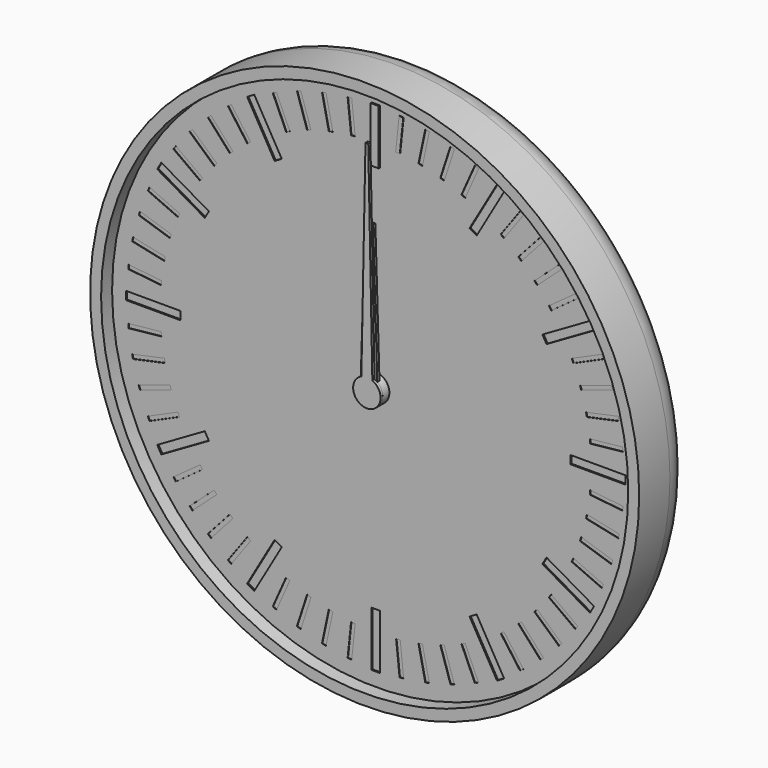
from build123d import *

# Parameters (mm, degrees)
F0_R      = 100
F1_DEPTH  = 24
F2_R      = 10
F3_T      = -4
F4_R      = 5
F4_R_2    = 3
F5_DEPTH  = 2
F6_DEPTH  = 19
F7_DEPTH  = 8
F9_DEPTH  = 4
F11_DEPTH = 4
F12_R     = 5
F12_R_2   = 3
F13_DEPTH = 2
F14_R     = 3
F15_DEPTH = 4
F17_DEPTH = 4
F18_R     = 3
F19_DEPTH = 2
F20_R     = 98
F20_R_2   = 5
F21_DEPTH = 1
F23_R     = 5
F23_R_2   = 3
F24_DEPTH = 2
F25_W     = 3
F25_H     = 20
F25_W_2   = 20
F25_H_2   = 3
F26_DEPTH = 0.5
F27_W     = 1.5
F27_H     = 12
F27_W_2   = 12
F27_H_2   = 1.5
F28_DEPTH = 0.2
F29_DEPTH = 1
F30_DEPTH = 0.4
F31_R     = 5
F31_R_2   = 3
F32_DEPTH = 5
F33_R     = 3
F34_DEPTH = 1
F36_DEPTH = 1


with BuildPart() as f1:
    # F0 (on Front) → F1 (new body)
    with BuildSketch(Plane.XZ):
        Circle(F0_R)
    extrude(amount=F1_DEPTH)

    # F2
    f2_edges = [f1.edges().sort_by_distance(p)[0] for p in [
        (-100, 0, 0),
    ]]
    fillet(f2_edges, radius=F2_R)

    # F3
    f3_openings = [f1.faces().sort_by_distance(p)[0] for p in [
        (0, -24, 0),
    ]]
    offset(amount=F3_T, openings=f3_openings)

    # F4 (on face) → F5 (join)
    with BuildSketch(Plane.XZ.offset(4)):
        with Locations((40, 0)):
            Circle(F4_R)
        with Locations((40, 0)):
            Circle(F4_R_2, mode=Mode.SUBTRACT)
        Circle(F4_R)
        Circle(F4_R_2, mode=Mode.SUBTRACT)
    extrude(amount=F5_DEPTH)


with BuildPart() as f6:
    # F6 (new): a face of the model
    f6_faces = [f1.part.faces().sort_by_distance(p)[0] for p in [
        (0, -4, 0),
    ]]
    extrude(f6_faces, amount=F6_DEPTH)

    # F8 (on face) → F9 (join)
    with BuildSketch(Plane.XZ.offset(6)):
        with BuildLine():
            ThreePointArc((9.2729637667, -1.3794085621), (9.3494561423, -0.6915886375), (9.375, 0))
            ThreePointArc((9.375, 0), (9.3494561423, 0.6915886375), (9.2729637667, 1.3794085621))
            ThreePointArc((9.2729637667, 1.3794085621), (8.9161548403, 2.8970343223), (8.3127812852, 4.3345463782))
            ThreePointArc((8.3127812852, 4.3345463782), (7.5845343223, 5.5104867402), (6.6911892658, 6.566476316))
            ThreePointArc((6.6911892658, 6.566476316), (5.5104867402, 7.5845343223), (4.1773988938, 8.3928519278))
            ThreePointArc((4.1773988938, 8.3928519278), (2.8970343223, 8.9161548403), (1.5536078905, 9.2453733036))
            ThreePointArc((1.5536078905, 9.2453733036), (0, 9.375), (-1.5536078905, 9.2453733036))
            ThreePointArc((-1.5536078905, 9.2453733036), (-2.8970343223, 8.9161548403), (-4.1773988938, 8.3928519278))
            ThreePointArc((-4.1773988938, 8.3928519278), (-5.5104867402, 7.5845343223), (-6.6911892658, 6.566476316))
            ThreePointArc((-6.6911892658, 6.566476316), (-7.5845343223, 5.5104867402), (-8.3127812852, 4.3345463782))
            ThreePointArc((-8.3127812852, 4.3345463782), (-8.9161548403, 2.8970343223), (-9.2729637667, 1.3794085621))
            ThreePointArc((-9.2729637667, 1.3794085621), (-9.375, 0), (-9.2729637667, -1.3794085621))
            ThreePointArc((-9.2729637667, -1.3794085621), (-8.9161548403, -2.8970343223), (-8.3127812852, -4.3345463782))
            ThreePointArc((-8.3127812852, -4.3345463782), (-7.5845343223, -5.5104867402), (-6.6911892658, -6.566476316))
            ThreePointArc((-6.6911892658, -6.566476316), (-5.5104867402, -7.5845343223), (-4.1773988938, -8.3928519278))
            ThreePointArc((-4.1773988938, -8.3928519278), (-2.8970343223, -8.9161548403), (-1.5536078905, -9.2453733036))
            ThreePointArc((-1.5536078905, -9.2453733036), (0, -9.375), (1.5536078905, -9.2453733036))
            ThreePointArc((1.5536078905, -9.2453733036), (2.8970343223, -8.9161548403), (4.1773988938, -8.3928519278))
            ThreePointArc((4.1773988938, -8.3928519278), (5.5104867402, -7.5845343223), (6.6911892658, -6.566476316))
            ThreePointArc((6.6911892658, -6.566476316), (7.5845343223, -5.5104867402), (8.3127812852, -4.3345463782))
            ThreePointArc((8.3127812852, -4.3345463782), (8.9161548403, -2.8970343223), (9.2729637667, -1.3794085621))
        make_face()
        with BuildLine():
            ThreePointArc((8.3127812852, 4.3345463782), (8.9161548403, 2.8970343223), (9.2729637667, 1.3794085621))
            Line((9.2729637667, 1.3794085621), (11.1823199426, 2.3946312492))
            Line((11.1823199426, 2.3946312492), (10.8182678729, 3.515068311))
            Line((10.8182678729, 3.515068311), (10.4542158031, 4.6355053728))
            Line((10.4542158031, 4.6355053728), (8.3127812852, 4.3345463782))
        make_face()
        with BuildLine():
            Line((11.1823199426, -2.3946312492), (9.2729637667, -1.3794085621))
            ThreePointArc((9.2729637667, -1.3794085621), (8.9161548403, -2.8970343223), (8.3127812852, -4.3345463782))
            Line((8.3127812852, -4.3345463782), (10.4542158031, -4.6355053728))
            Line((10.4542158031, -4.6355053728), (10.8182678729, -3.515068311))
            Line((10.8182678729, -3.515068311), (11.1823199426, -2.3946312492))
        make_face()
        with BuildLine():
            ThreePointArc((4.1773988938, 8.3928519278), (5.5104867402, 7.5845343223), (6.6911892658, 6.566476316))
            Line((6.6911892658, 6.566476316), (7.6391579371, 8.5101001246))
            Line((7.6391579371, 8.5101001246), (6.6860572448, 9.202568311))
            Line((6.6860572448, 9.202568311), (5.7329565525, 9.8950364974))
            Line((5.7329565525, 9.8950364974), (4.1773988938, 8.3928519278))
        make_face()
        with BuildLine():
            Line((7.6391579371, -8.5101001246), (6.6911892658, -6.566476316))
            ThreePointArc((6.6911892658, -6.566476316), (5.5104867402, -7.5845343223), (4.1773988938, -8.3928519278))
            Line((4.1773988938, -8.3928519278), (5.7329565525, -9.8950364974))
            Line((5.7329565525, -9.8950364974), (6.6860572448, -9.202568311))
            Line((6.6860572448, -9.202568311), (7.6391579371, -8.5101001246))
        make_face()
        with BuildLine():
            ThreePointArc((-1.5536078905, 9.2453733036), (0, 9.375), (1.5536078905, 9.2453733036))
            Line((1.5536078905, 9.2453733036), (1.1780972451, 11.375))
            Line((1.1780972451, 11.375), (0, 11.375))
            Line((0, 11.375), (-1.1780972451, 11.375))
            Line((-1.1780972451, 11.375), (-1.5536078905, 9.2453733036))
        make_face()
        with BuildLine():
            Line((1.1780972451, -11.375), (1.5536078905, -9.2453733036))
            ThreePointArc((1.5536078905, -9.2453733036), (0, -9.375), (-1.5536078905, -9.2453733036))
            Line((-1.5536078905, -9.2453733036), (-1.1780972451, -11.375))
            Line((-1.1780972451, -11.375), (0, -11.375))
            Line((0, -11.375), (1.1780972451, -11.375))
        make_face()
        with BuildLine():
            ThreePointArc((-6.6911892658, 6.566476316), (-5.5104867402, 7.5845343223), (-4.1773988938, 8.3928519278))
            Line((-4.1773988938, 8.3928519278), (-5.7329565525, 9.8950364974))
            Line((-5.7329565525, 9.8950364974), (-6.6860572448, 9.202568311))
            Line((-6.6860572448, 9.202568311), (-7.6391579371, 8.5101001246))
            Line((-7.6391579371, 8.5101001246), (-6.6911892658, 6.566476316))
        make_face()
        with BuildLine():
            Line((-5.7329565525, -9.8950364974), (-4.1773988938, -8.3928519278))
            ThreePointArc((-4.1773988938, -8.3928519278), (-5.5104867402, -7.5845343223), (-6.6911892658, -6.566476316))
            Line((-6.6911892658, -6.566476316), (-7.6391579371, -8.5101001246))
            Line((-7.6391579371, -8.5101001246), (-6.6860572448, -9.202568311))
            Line((-6.6860572448, -9.202568311), (-5.7329565525, -9.8950364974))
        make_face()
        with BuildLine():
            ThreePointArc((-9.2729637667, 1.3794085621), (-8.9161548403, 2.8970343223), (-8.3127812852, 4.3345463782))
            Line((-8.3127812852, 4.3345463782), (-10.4542158031, 4.6355053728))
            Line((-10.4542158031, 4.6355053728), (-10.8182678729, 3.515068311))
            Line((-10.8182678729, 3.515068311), (-11.1823199426, 2.3946312492))
            Line((-11.1823199426, 2.3946312492), (-9.2729637667, 1.3794085621))
        make_face()
        with BuildLine():
            Line((-10.4542158031, -4.6355053728), (-8.3127812852, -4.3345463782))
            ThreePointArc((-8.3127812852, -4.3345463782), (-8.9161548403, -2.8970343223), (-9.2729637667, -1.3794085621))
            Line((-9.2729637667, -1.3794085621), (-11.1823199426, -2.3946312492))
            Line((-11.1823199426, -2.3946312492), (-10.8182678729, -3.515068311))
            Line((-10.8182678729, -3.515068311), (-10.4542158031, -4.6355053728))
        make_face()
    extrude(amount=F9_DEPTH)

    # F35 (on face) → F36 (join)
    with BuildSketch(Plane.XZ.offset(23)):
        with BuildLine():
            ThreePointArc((-2, 4.582575695), (-2.7386127875, -4.1833001327), (5, 0))
            ThreePointArc((5, 0), (4.1833001327, 2.7386127875), (2, 4.582575695))
            ThreePointArc((2, 4.582575695), (0, 5), (-2, 4.582575695))
        make_face()
        with BuildLine():
            ThreePointArc((-2, 4.582575695), (0, 5), (2, 4.582575695))
            Line((2, 4.582575695), (0.5, 80))
            Line((0.5, 80), (0, 80))
            Line((0, 80), (-0.5, 80))
            Line((-0.5, 80), (-2, 4.582575695))
        make_face()
    extrude(amount=-F36_DEPTH)


with BuildPart() as f7:
    # F7 (new): a face of the model
    f7_faces = [f1.part.faces().sort_by_distance(p)[0] for p in [
        (40, -4, 0),
    ]]
    extrude(f7_faces, amount=F7_DEPTH)

    # F10 (on face) → F11 (join)
    with BuildSketch(Plane.XZ.offset(6)):
        with BuildLine():
            ThreePointArc((68.0829066802, -1.5381733945), (68.1144747006, -0.7693746225), (68.125, 0))
            ThreePointArc((68.125, 0), (68.1144747006, 0.7693746225), (68.0829066802, 1.5381733945))
            ThreePointArc((68.0829066802, 1.5381733945), (67.9709283072, 2.9398630294), (67.7890320221, 4.3342039956))
            ThreePointArc((67.7890320221, 4.3342039956), (67.5104012706, 5.8475163042), (67.1494235596, 7.3433252263))
            ThreePointArc((67.1494235596, 7.3433252263), (66.7484645208, 8.6911029668), (66.280643318, 10.0171558733))
            ThreePointArc((66.280643318, 10.0171558733), (65.6934659962, 11.4394680865), (65.0293803521, 12.8275385085))
            ThreePointArc((65.0293803521, 12.8275385085), (64.3569644814, 14.0625), (63.6236643925, 15.2623099717))
            ThreePointArc((63.6236643925, 15.2623099717), (62.7536029668, 16.5314602207), (61.815433119, 17.7511268046))
            ThreePointArc((61.815433119, 17.7511268046), (60.9009482166, 18.8192983038), (59.934217974, 19.8404278876))
            ThreePointArc((59.934217974, 19.8404278876), (58.8192983038, 20.9009482166), (57.6480467764, 21.8989056799))
            ThreePointArc((57.6480467764, 21.8989056799), (56.5314602207, 22.7536029668), (55.3735505752, 23.5514238999))
            ThreePointArc((55.3735505752, 23.5514238999), (54.0625, 24.3569644814), (52.709356105, 25.0895972944))
            ThreePointArc((52.709356105, 25.0895972944), (51.4394680865, 25.6934659962), (50.1409852457, 26.2331096755))
            ThreePointArc((50.1409852457, 26.2331096755), (48.6911029668, 26.7484645208), (47.2152055856, 27.1837531139))
            ThreePointArc((47.2152055856, 27.1837531139), (45.8475163042, 27.5104012706), (44.4652101991, 27.7682826779))
            ThreePointArc((44.4652101991, 27.7682826779), (42.9398630294, 27.9709283072), (41.4057159597, 28.0898484802))
            ThreePointArc((41.4057159597, 28.0898484802), (40, 28.125), (38.5942840403, 28.0898484802))
            ThreePointArc((38.5942840403, 28.0898484802), (37.0601369706, 27.9709283072), (35.5347898009, 27.7682826779))
            ThreePointArc((35.5347898009, 27.7682826779), (34.1524836958, 27.5104012706), (32.7847944144, 27.1837531139))
            ThreePointArc((32.7847944144, 27.1837531139), (31.3088970332, 26.7484645208), (29.8590147543, 26.2331096755))
            ThreePointArc((29.8590147543, 26.2331096755), (28.5605319135, 25.6934659962), (27.290643895, 25.0895972944))
            ThreePointArc((27.290643895, 25.0895972944), (25.9375, 24.3569644814), (24.6264494248, 23.5514238999))
            ThreePointArc((24.6264494248, 23.5514238999), (23.4685397793, 22.7536029668), (22.3519532236, 21.8989056799))
            ThreePointArc((22.3519532236, 21.8989056799), (21.1807016962, 20.9009482166), (20.065782026, 19.8404278876))
            ThreePointArc((20.065782026, 19.8404278876), (19.0990517834, 18.8192983038), (18.184566881, 17.7511268046))
            ThreePointArc((18.184566881, 17.7511268046), (17.2463970332, 16.5314602207), (16.3763356075, 15.2623099717))
            ThreePointArc((16.3763356075, 15.2623099717), (15.6430355186, 14.0625), (14.9706196479, 12.8275385085))
            ThreePointArc((14.9706196479, 12.8275385085), (14.3065340038, 11.4394680865), (13.719356682, 10.0171558733))
            ThreePointArc((13.719356682, 10.0171558733), (13.2515354792, 8.6911029668), (12.8505764404, 7.3433252263))
            ThreePointArc((12.8505764404, 7.3433252263), (12.4895987294, 5.8475163042), (12.2109679779, 4.3342039956))
            ThreePointArc((12.2109679779, 4.3342039956), (12.0290716928, 2.9398630294), (11.9170933198, 1.5381733945))
            ThreePointArc((11.9170933198, 1.5381733945), (11.875, 0), (11.9170933198, -1.5381733945))
            ThreePointArc((11.9170933198, -1.5381733945), (12.0290716928, -2.9398630294), (12.2109679779, -4.3342039956))
            ThreePointArc((12.2109679779, -4.3342039956), (12.4895987294, -5.8475163042), (12.8505764404, -7.3433252263))
            ThreePointArc((12.8505764404, -7.3433252263), (13.2515354792, -8.6911029668), (13.719356682, -10.0171558733))
            ThreePointArc((13.719356682, -10.0171558733), (14.3065340038, -11.4394680865), (14.9706196479, -12.8275385085))
            ThreePointArc((14.9706196479, -12.8275385085), (15.6430355186, -14.0625), (16.3763356075, -15.2623099717))
            ThreePointArc((16.3763356075, -15.2623099717), (17.2463970332, -16.5314602207), (18.184566881, -17.7511268046))
            ThreePointArc((18.184566881, -17.7511268046), (19.0990517834, -18.8192983038), (20.065782026, -19.8404278876))
            ThreePointArc((20.065782026, -19.8404278876), (21.1807016962, -20.9009482166), (22.3519532236, -21.8989056799))
            ThreePointArc((22.3519532236, -21.8989056799), (23.4685397793, -22.7536029668), (24.6264494248, -23.5514238999))
            ThreePointArc((24.6264494248, -23.5514238999), (25.9375, -24.3569644814), (27.290643895, -25.0895972944))
            ThreePointArc((27.290643895, -25.0895972944), (28.5605319135, -25.6934659962), (29.8590147543, -26.2331096755))
            ThreePointArc((29.8590147543, -26.2331096755), (31.3088970332, -26.7484645208), (32.7847944144, -27.1837531139))
            ThreePointArc((32.7847944144, -27.1837531139), (34.1524836958, -27.5104012706), (35.5347898009, -27.7682826779))
            ThreePointArc((35.5347898009, -27.7682826779), (37.0601369706, -27.9709283072), (38.5942840403, -28.0898484802))
            ThreePointArc((38.5942840403, -28.0898484802), (40, -28.125), (41.4057159597, -28.0898484802))
            ThreePointArc((41.4057159597, -28.0898484802), (42.9398630294, -27.9709283072), (44.4652101991, -27.7682826779))
            ThreePointArc((44.4652101991, -27.7682826779), (45.8475163042, -27.5104012706), (47.2152055856, -27.1837531139))
            ThreePointArc((47.2152055856, -27.1837531139), (48.6911029668, -26.7484645208), (50.1409852457, -26.2331096755))
            ThreePointArc((50.1409852457, -26.2331096755), (51.4394680865, -25.6934659962), (52.709356105, -25.0895972944))
            ThreePointArc((52.709356105, -25.0895972944), (54.0625, -24.3569644814), (55.3735505752, -23.5514238999))
            ThreePointArc((55.3735505752, -23.5514238999), (56.5314602207, -22.7536029668), (57.6480467764, -21.8989056799))
            ThreePointArc((57.6480467764, -21.8989056799), (58.8192983038, -20.9009482166), (59.934217974, -19.8404278876))
            ThreePointArc((59.934217974, -19.8404278876), (60.9009482166, -18.8192983038), (61.815433119, -17.7511268046))
            ThreePointArc((61.815433119, -17.7511268046), (62.7536029668, -16.5314602207), (63.6236643925, -15.2623099717))
            ThreePointArc((63.6236643925, -15.2623099717), (64.3569644814, -14.0625), (65.0293803521, -12.8275385085))
            ThreePointArc((65.0293803521, -12.8275385085), (65.6934659962, -11.4394680865), (66.280643318, -10.0171558733))
            ThreePointArc((66.280643318, -10.0171558733), (66.7484645208, -8.6911029668), (67.1494235596, -7.3433252263))
            ThreePointArc((67.1494235596, -7.3433252263), (67.5104012706, -5.8475163042), (67.7890320221, -4.3342039956))
            ThreePointArc((67.7890320221, -4.3342039956), (67.9709283072, -2.9398630294), (68.0829066802, -1.5381733945))
        make_face()
        with BuildLine():
            ThreePointArc((68.0829066802, 1.5381733945), (68.1144747006, 0.7693746225), (68.125, 0))
            ThreePointArc((68.125, 0), (68.1144747006, -0.7693746225), (68.0829066802, -1.5381733945))
            Line((68.0829066802, -1.5381733945), (70.125, -1.1780972451))
            Line((70.125, -1.1780972451), (70.125, 0))
            Line((70.125, 0), (70.125, 1.1780972451))
            Line((70.125, 1.1780972451), (68.0829066802, 1.5381733945))
        make_face()
        with BuildLine():
            ThreePointArc((67.1494235596, 7.3433252263), (67.5104012706, 5.8475163042), (67.7890320221, 4.3342039956))
            Line((67.7890320221, 4.3342039956), (69.7116366623, 5.1109866922))
            Line((69.7116366623, 5.1109866922), (69.4666964721, 6.2633396859))
            Line((69.4666964721, 6.2633396859), (69.2217562819, 7.4156926796))
            Line((69.2217562819, 7.4156926796), (67.1494235596, 7.3433252263))
        make_face()
        with BuildLine():
            Line((69.7116366623, -5.1109866922), (67.7890320221, -4.3342039956))
            ThreePointArc((67.7890320221, -4.3342039956), (67.5104012706, -5.8475163042), (67.1494235596, -7.3433252263))
            Line((67.1494235596, -7.3433252263), (69.2217562819, -7.4156926796))
            Line((69.2217562819, -7.4156926796), (69.4666964721, -6.2633396859))
            Line((69.4666964721, -6.2633396859), (69.7116366623, -5.1109866922))
        make_face()
        with BuildLine():
            ThreePointArc((65.0293803521, 12.8275385085), (65.6934659962, 11.4394680865), (66.280643318, 10.0171558733))
            Line((66.280643318, 10.0171558733), (67.9997322302, 11.1766959857))
            Line((67.9997322302, 11.1766959857), (67.5205569115, 12.2529413727))
            Line((67.5205569115, 12.2529413727), (67.0413815928, 13.3291867596))
            Line((67.0413815928, 13.3291867596), (65.0293803521, 12.8275385085))
        make_face()
        with BuildLine():
            Line((67.9997322302, -11.1766959857), (66.280643318, -10.0171558733))
            ThreePointArc((66.280643318, -10.0171558733), (65.6934659962, -11.4394680865), (65.0293803521, -12.8275385085))
            Line((65.0293803521, -12.8275385085), (67.0413815928, -13.3291867596))
            Line((67.0413815928, -13.3291867596), (67.5205569115, -12.2529413727))
            Line((67.5205569115, -12.2529413727), (67.9997322302, -11.1766959857))
        make_face()
        with BuildLine():
            ThreePointArc((61.815433119, 17.7511268046), (62.7536029668, 16.5314602207), (63.6236643925, 15.2623099717))
            Line((63.6236643925, 15.2623099717), (65.064105142, 16.753930033))
            Line((65.064105142, 16.753930033), (64.3716369555, 17.7070307253))
            Line((64.3716369555, 17.7070307253), (63.6791687691, 18.6601314176))
            Line((63.6791687691, 18.6601314176), (61.815433119, 17.7511268046))
        make_face()
        with BuildLine():
            Line((65.064105142, -16.753930033), (63.6236643925, -15.2623099717))
            ThreePointArc((63.6236643925, -15.2623099717), (62.7536029668, -16.5314602207), (61.815433119, -17.7511268046))
            Line((61.815433119, -17.7511268046), (63.6791687691, -18.6601314176))
            Line((63.6791687691, -18.6601314176), (64.3716369555, -17.7070307253))
            Line((64.3716369555, -17.7070307253), (65.064105142, -16.753930033))
        make_face()
        with BuildLine():
            ThreePointArc((57.6480467764, 21.8989056799), (58.8192983038, 20.9009482166), (59.934217974, 19.8404278876))
            Line((59.934217974, 19.8404278876), (61.0330563882, 21.5989369435))
            Line((61.0330563882, 21.5989369435), (60.1575595166, 22.3872378675))
            Line((60.1575595166, 22.3872378675), (59.282062645, 23.1755387915))
            Line((59.282062645, 23.1755387915), (57.6480467764, 21.8989056799))
        make_face()
        with BuildLine():
            Line((61.0330563882, -21.5989369435), (59.934217974, -19.8404278876))
            ThreePointArc((59.934217974, -19.8404278876), (58.8192983038, -20.9009482166), (57.6480467764, -21.8989056799))
            Line((57.6480467764, -21.8989056799), (59.282062645, -23.1755387915))
            Line((59.282062645, -23.1755387915), (60.1575595166, -22.3872378675))
            Line((60.1575595166, -22.3872378675), (61.0330563882, -21.5989369435))
        make_face()
        with BuildLine():
            ThreePointArc((52.709356105, 25.0895972944), (54.0625, 24.3569644814), (55.3735505752, 23.5514238999))
            Line((55.3735505752, 23.5514238999), (56.0827621424, 25.4999666665))
            Line((56.0827621424, 25.4999666665), (55.0625, 26.089015289))
            Line((55.0625, 26.089015289), (54.0422378576, 26.6780639116))
            Line((54.0422378576, 26.6780639116), (52.709356105, 25.0895972944))
        make_face()
        with BuildLine():
            Line((56.0827621424, -25.4999666665), (55.3735505752, -23.5514238999))
            ThreePointArc((55.3735505752, -23.5514238999), (54.0625, -24.3569644814), (52.709356105, -25.0895972944))
            Line((52.709356105, -25.0895972944), (54.0422378576, -26.6780639116))
            Line((54.0422378576, -26.6780639116), (55.0625, -26.089015289))
            Line((55.0625, -26.089015289), (56.0827621424, -25.4999666665))
        make_face()
        with BuildLine():
            ThreePointArc((47.2152055856, 27.1837531139), (48.6911029668, 26.7484645208), (50.1409852457, 26.2331096755))
            Line((50.1409852457, 26.2331096755), (50.4295740173, 28.2865254836))
            Line((50.4295740173, 28.2865254836), (49.3091369555, 28.6505775534))
            Line((49.3091369555, 28.6505775534), (48.1886998938, 29.0146296232))
            Line((48.1886998938, 29.0146296232), (47.2152055856, 27.1837531139))
        make_face()
        with BuildLine():
            Line((50.4295740173, -28.2865254836), (50.1409852457, -26.2331096755))
            ThreePointArc((50.1409852457, -26.2331096755), (48.6911029668, -26.7484645208), (47.2152055856, -27.1837531139))
            Line((47.2152055856, -27.1837531139), (48.1886998938, -29.0146296232))
            Line((48.1886998938, -29.0146296232), (49.3091369555, -28.6505775534))
            Line((49.3091369555, -28.6505775534), (50.4295740173, -28.2865254836))
        make_face()
        with BuildLine():
            ThreePointArc((41.4057159597, 28.0898484802), (42.9398630294, 27.9709283072), (44.4652101991, 27.7682826779))
            Line((44.4652101991, 27.7682826779), (44.3205634611, 29.8368274034))
            Line((44.3205634611, 29.8368274034), (43.1489199559, 29.959972098))
            Line((43.1489199559, 29.959972098), (41.9772764508, 30.0831167926))
            Line((41.9772764508, 30.0831167926), (41.4057159597, 28.0898484802))
        make_face()
        with BuildLine():
            Line((44.3205634611, -29.8368274034), (44.4652101991, -27.7682826779))
            ThreePointArc((44.4652101991, -27.7682826779), (42.9398630294, -27.9709283072), (41.4057159597, -28.0898484802))
            Line((41.4057159597, -28.0898484802), (41.9772764508, -30.0831167926))
            Line((41.9772764508, -30.0831167926), (43.1489199559, -29.959972098))
            Line((43.1489199559, -29.959972098), (44.3205634611, -29.8368274034))
        make_face()
        with BuildLine():
            ThreePointArc((35.5347898009, 27.7682826779), (37.0601369706, 27.9709283072), (38.5942840403, 28.0898484802))
            Line((38.5942840403, 28.0898484802), (38.0227235492, 30.0831167926))
            Line((38.0227235492, 30.0831167926), (36.8510800441, 29.959972098))
            Line((36.8510800441, 29.959972098), (35.6794365389, 29.8368274034))
            Line((35.6794365389, 29.8368274034), (35.5347898009, 27.7682826779))
        make_face()
        with BuildLine():
            Line((38.0227235492, -30.0831167926), (38.5942840403, -28.0898484802))
            ThreePointArc((38.5942840403, -28.0898484802), (37.0601369706, -27.9709283072), (35.5347898009, -27.7682826779))
            Line((35.5347898009, -27.7682826779), (35.6794365389, -29.8368274034))
            Line((35.6794365389, -29.8368274034), (36.8510800441, -29.959972098))
            Line((36.8510800441, -29.959972098), (38.0227235492, -30.0831167926))
        make_face()
        with BuildLine():
            ThreePointArc((29.8590147543, 26.2331096755), (31.3088970332, 26.7484645208), (32.7847944144, 27.1837531139))
            Line((32.7847944144, 27.1837531139), (31.8113001062, 29.0146296232))
            Line((31.8113001062, 29.0146296232), (30.6908630445, 28.6505775534))
            Line((30.6908630445, 28.6505775534), (29.5704259827, 28.2865254836))
            Line((29.5704259827, 28.2865254836), (29.8590147543, 26.2331096755))
        make_face()
        with BuildLine():
            Line((31.8113001062, -29.0146296232), (32.7847944144, -27.1837531139))
            ThreePointArc((32.7847944144, -27.1837531139), (31.3088970332, -26.7484645208), (29.8590147543, -26.2331096755))
            Line((29.8590147543, -26.2331096755), (29.5704259827, -28.2865254836))
            Line((29.5704259827, -28.2865254836), (30.6908630445, -28.6505775534))
            Line((30.6908630445, -28.6505775534), (31.8113001062, -29.0146296232))
        make_face()
        with BuildLine():
            ThreePointArc((24.6264494248, 23.5514238999), (25.9375, 24.3569644814), (27.290643895, 25.0895972944))
            Line((27.290643895, 25.0895972944), (25.9577621424, 26.6780639116))
            Line((25.9577621424, 26.6780639116), (24.9375, 26.089015289))
            Line((24.9375, 26.089015289), (23.9172378576, 25.4999666665))
            Line((23.9172378576, 25.4999666665), (24.6264494248, 23.5514238999))
        make_face()
        with BuildLine():
            Line((25.9577621424, -26.6780639116), (27.290643895, -25.0895972944))
            ThreePointArc((27.290643895, -25.0895972944), (25.9375, -24.3569644814), (24.6264494248, -23.5514238999))
            Line((24.6264494248, -23.5514238999), (23.9172378576, -25.4999666665))
            Line((23.9172378576, -25.4999666665), (24.9375, -26.089015289))
            Line((24.9375, -26.089015289), (25.9577621424, -26.6780639116))
        make_face()
        with BuildLine():
            ThreePointArc((20.065782026, 19.8404278876), (21.1807016962, 20.9009482166), (22.3519532236, 21.8989056799))
            Line((22.3519532236, 21.8989056799), (20.717937355, 23.1755387915))
            Line((20.717937355, 23.1755387915), (19.8424404834, 22.3872378675))
            Line((19.8424404834, 22.3872378675), (18.9669436118, 21.5989369435))
            Line((18.9669436118, 21.5989369435), (20.065782026, 19.8404278876))
        make_face()
        with BuildLine():
            Line((20.717937355, -23.1755387915), (22.3519532236, -21.8989056799))
            ThreePointArc((22.3519532236, -21.8989056799), (21.1807016962, -20.9009482166), (20.065782026, -19.8404278876))
            Line((20.065782026, -19.8404278876), (18.9669436118, -21.5989369435))
            Line((18.9669436118, -21.5989369435), (19.8424404834, -22.3872378675))
            Line((19.8424404834, -22.3872378675), (20.717937355, -23.1755387915))
        make_face()
        with BuildLine():
            ThreePointArc((16.3763356075, 15.2623099717), (17.2463970332, 16.5314602207), (18.184566881, 17.7511268046))
            Line((18.184566881, 17.7511268046), (16.3208312309, 18.6601314176))
            Line((16.3208312309, 18.6601314176), (15.6283630445, 17.7070307253))
            Line((15.6283630445, 17.7070307253), (14.935894858, 16.753930033))
            Line((14.935894858, 16.753930033), (16.3763356075, 15.2623099717))
        make_face()
        with BuildLine():
            Line((16.3208312309, -18.6601314176), (18.184566881, -17.7511268046))
            ThreePointArc((18.184566881, -17.7511268046), (17.2463970332, -16.5314602207), (16.3763356075, -15.2623099717))
            Line((16.3763356075, -15.2623099717), (14.935894858, -16.753930033))
            Line((14.935894858, -16.753930033), (15.6283630445, -17.7070307253))
            Line((15.6283630445, -17.7070307253), (16.3208312309, -18.6601314176))
        make_face()
        with BuildLine():
            ThreePointArc((13.719356682, 10.0171558733), (14.3065340038, 11.4394680865), (14.9706196479, 12.8275385085))
            Line((14.9706196479, 12.8275385085), (12.9586184072, 13.3291867596))
            Line((12.9586184072, 13.3291867596), (12.4794430885, 12.2529413727))
            Line((12.4794430885, 12.2529413727), (12.0002677698, 11.1766959857))
            Line((12.0002677698, 11.1766959857), (13.719356682, 10.0171558733))
        make_face()
        with BuildLine():
            Line((12.9586184072, -13.3291867596), (14.9706196479, -12.8275385085))
            ThreePointArc((14.9706196479, -12.8275385085), (14.3065340038, -11.4394680865), (13.719356682, -10.0171558733))
            Line((13.719356682, -10.0171558733), (12.0002677698, -11.1766959857))
            Line((12.0002677698, -11.1766959857), (12.4794430885, -12.2529413727))
            Line((12.4794430885, -12.2529413727), (12.9586184072, -13.3291867596))
        make_face()
        with BuildLine():
            ThreePointArc((12.2109679779, 4.3342039956), (12.4895987294, 5.8475163042), (12.8505764404, 7.3433252263))
            Line((12.8505764404, 7.3433252263), (10.7782437181, 7.4156926796))
            Line((10.7782437181, 7.4156926796), (10.5333035279, 6.2633396859))
            Line((10.5333035279, 6.2633396859), (10.2883633377, 5.1109866922))
            Line((10.2883633377, 5.1109866922), (12.2109679779, 4.3342039956))
        make_face()
        with BuildLine():
            Line((10.7782437181, -7.4156926796), (12.8505764404, -7.3433252263))
            ThreePointArc((12.8505764404, -7.3433252263), (12.4895987294, -5.8475163042), (12.2109679779, -4.3342039956))
            Line((12.2109679779, -4.3342039956), (10.2883633377, -5.1109866922))
            Line((10.2883633377, -5.1109866922), (10.5333035279, -6.2633396859))
            Line((10.5333035279, -6.2633396859), (10.7782437181, -7.4156926796))
        make_face()
        with BuildLine():
            ThreePointArc((11.9170933198, -1.5381733945), (11.875, 0), (11.9170933198, 1.5381733945))
            Line((11.9170933198, 1.5381733945), (9.875, 1.1780972451))
            Line((9.875, 1.1780972451), (9.875, 0))
            Line((9.875, 0), (9.875, -1.1780972451))
            Line((9.875, -1.1780972451), (11.9170933198, -1.5381733945))
        make_face()
    extrude(amount=F11_DEPTH)

    # F16 (on face) → F17 (join)
    with BuildSketch(Plane.XZ.offset(12)):
        with BuildLine():
            ThreePointArc((47.4288750323, -1.0304444454), (47.4821976298, -0.5164480894), (47.5, 0))
            ThreePointArc((47.5, 0), (47.4821976298, 0.5164480894), (47.4288750323, 1.0304444454))
            ThreePointArc((47.4288750323, 1.0304444454), (47.1329238722, 2.3176274578), (46.6157661985, 3.532936117))
            ThreePointArc((46.6157661985, 3.532936117), (46.0676274578, 4.4083893922), (45.4044061018, 5.2002302532))
            ThreePointArc((45.4044061018, 5.2002302532), (44.4083893922, 6.0676274578), (43.2756595386, 6.7468551628))
            ThreePointArc((43.2756595386, 6.7468551628), (42.3176274578, 7.1329238722), (41.3156377295, 7.3837048536))
            ThreePointArc((41.3156377295, 7.3837048536), (40, 7.5), (38.6843622705, 7.3837048536))
            ThreePointArc((38.6843622705, 7.3837048536), (37.6823725422, 7.1329238722), (36.7243404614, 6.7468551628))
            ThreePointArc((36.7243404614, 6.7468551628), (35.5916106078, 6.0676274578), (34.5955938982, 5.2002302532))
            ThreePointArc((34.5955938982, 5.2002302532), (33.9323725422, 4.4083893922), (33.3842338015, 3.532936117))
            ThreePointArc((33.3842338015, 3.532936117), (32.8670761278, 2.3176274578), (32.5711249677, 1.0304444454))
            ThreePointArc((32.5711249677, 1.0304444454), (32.5, 0), (32.5711249677, -1.0304444454))
            ThreePointArc((32.5711249677, -1.0304444454), (32.8670761278, -2.3176274578), (33.3842338015, -3.532936117))
            ThreePointArc((33.3842338015, -3.532936117), (33.9323725422, -4.4083893922), (34.5955938982, -5.2002302532))
            ThreePointArc((34.5955938982, -5.2002302532), (35.5916106078, -6.0676274578), (36.7243404614, -6.7468551628))
            ThreePointArc((36.7243404614, -6.7468551628), (37.6823725422, -7.1329238722), (38.6843622705, -7.3837048536))
            ThreePointArc((38.6843622705, -7.3837048536), (40, -7.5), (41.3156377295, -7.3837048536))
            ThreePointArc((41.3156377295, -7.3837048536), (42.3176274578, -7.1329238722), (43.2756595386, -6.7468551628))
            ThreePointArc((43.2756595386, -6.7468551628), (44.4083893922, -6.0676274578), (45.4044061018, -5.2002302532))
            ThreePointArc((45.4044061018, -5.2002302532), (46.0676274578, -4.4083893922), (46.6157661985, -3.532936117))
            ThreePointArc((46.6157661985, -3.532936117), (47.1329238722, -2.3176274578), (47.4288750323, -1.0304444454))
        make_face()
        with BuildLine():
            ThreePointArc((46.6157661985, 3.532936117), (47.1329238722, 2.3176274578), (47.4288750323, 1.0304444454))
            Line((47.4288750323, 1.0304444454), (49.3262785606, 2.0393117971))
            Line((49.3262785606, 2.0393117971), (48.743795249, 3.832011096))
            Line((48.743795249, 3.832011096), (46.6157661985, 3.532936117))
        make_face()
        with BuildLine():
            Line((49.3262785606, -2.0393117971), (47.4288750323, -1.0304444454))
            ThreePointArc((47.4288750323, -1.0304444454), (47.1329238722, -2.3176274578), (46.6157661985, -3.532936117))
            Line((46.6157661985, -3.532936117), (48.743795249, -3.832011096))
            Line((48.743795249, -3.832011096), (49.3262785606, -2.0393117971))
        make_face()
        with BuildLine():
            ThreePointArc((43.2756595386, 6.7468551628), (44.4083893922, 6.0676274578), (45.4044061018, 5.2002302532))
            Line((45.4044061018, 5.2002302532), (46.3464404506, 7.1316868974))
            Line((46.3464404506, 7.1316868974), (44.8214793429, 8.2396359957))
            Line((44.8214793429, 8.2396359957), (43.2756595386, 6.7468551628))
        make_face()
        with BuildLine():
            Line((46.3464404506, -7.1316868974), (45.4044061018, -5.2002302532))
            ThreePointArc((45.4044061018, -5.2002302532), (44.4083893922, -6.0676274578), (43.2756595386, -6.7468551628))
            Line((43.2756595386, -6.7468551628), (44.8214793429, -8.2396359957))
            Line((44.8214793429, -8.2396359957), (46.3464404506, -7.1316868974))
        make_face()
        with BuildLine():
            ThreePointArc((38.6843622705, 7.3837048536), (40, 7.5), (41.3156377295, 7.3837048536))
            Line((41.3156377295, 7.3837048536), (40.9424777961, 9.5))
            Line((40.9424777961, 9.5), (39.0575222039, 9.5))
            Line((39.0575222039, 9.5), (38.6843622705, 7.3837048536))
        make_face()
        with BuildLine():
            Line((40.9424777961, -9.5), (41.3156377295, -7.3837048536))
            ThreePointArc((41.3156377295, -7.3837048536), (40, -7.5), (38.6843622705, -7.3837048536))
            Line((38.6843622705, -7.3837048536), (39.0575222039, -9.5))
            Line((39.0575222039, -9.5), (40.9424777961, -9.5))
        make_face()
        with BuildLine():
            ThreePointArc((34.5955938982, 5.2002302532), (35.5916106078, 6.0676274578), (36.7243404614, 6.7468551628))
            Line((36.7243404614, 6.7468551628), (35.1785206571, 8.2396359957))
            Line((35.1785206571, 8.2396359957), (33.6535595494, 7.1316868974))
            Line((33.6535595494, 7.1316868974), (34.5955938982, 5.2002302532))
        make_face()
        with BuildLine():
            Line((35.1785206571, -8.2396359957), (36.7243404614, -6.7468551628))
            ThreePointArc((36.7243404614, -6.7468551628), (35.5916106078, -6.0676274578), (34.5955938982, -5.2002302532))
            Line((34.5955938982, -5.2002302532), (33.6535595494, -7.1316868974))
            Line((33.6535595494, -7.1316868974), (35.1785206571, -8.2396359957))
        make_face()
        with BuildLine():
            ThreePointArc((32.5711249677, 1.0304444454), (32.8670761278, 2.3176274578), (33.3842338015, 3.532936117))
            Line((33.3842338015, 3.532936117), (31.256204751, 3.832011096))
            Line((31.256204751, 3.832011096), (30.6737214394, 2.0393117971))
            Line((30.6737214394, 2.0393117971), (32.5711249677, 1.0304444454))
        make_face()
        with BuildLine():
            Line((31.256204751, -3.832011096), (33.3842338015, -3.532936117))
            ThreePointArc((33.3842338015, -3.532936117), (32.8670761278, -2.3176274578), (32.5711249677, -1.0304444454))
            Line((32.5711249677, -1.0304444454), (30.6737214394, -2.0393117971))
            Line((30.6737214394, -2.0393117971), (31.256204751, -3.832011096))
        make_face()
    extrude(amount=F17_DEPTH)

    # F18 (on face) → F19 (join)
    with BuildSketch(Plane.XZ.offset(16)):
        with Locations((40, 0)):
            Circle(F18_R)
    extrude(amount=F19_DEPTH)


with BuildPart() as f13:
    # F12 (on face) → F13 (new body)
    with BuildSketch(Plane.XZ.offset(10)):
        Circle(F12_R)
        Circle(F12_R_2, mode=Mode.SUBTRACT)
    extrude(amount=F13_DEPTH)

    # F14 (on face) → F15 (join)
    with BuildSketch(Plane.XZ.offset(12)):
        with BuildLine():
            ThreePointArc((29.9718156995, -1.3001014101), (29.9929530972, -0.6502034357), (30, 0))
            ThreePointArc((30, 0), (29.9929530972, 0.6502034357), (29.9718156995, 1.3001014101))
            ThreePointArc((29.9718156995, 1.3001014101), (29.907520012, 2.3537728718), (29.8061935814, 3.4045299509))
            ThreePointArc((29.8061935814, 3.4045299509), (29.6306502179, 4.6930339512), (29.3994322443, 5.9727199596))
            ThreePointArc((29.3994322443, 5.9727199596), (29.1710976119, 7.0033609157), (28.9066440563, 8.0253304855))
            ThreePointArc((28.9066440563, 8.0253304855), (28.5316954889, 9.2705098312), (28.1031371961, 10.4982703213))
            ThreePointArc((28.1031371961, 10.4982703213), (27.7163859753, 11.480502971), (27.2953170189, 12.448520749))
            ThreePointArc((27.2953170189, 12.448520749), (26.7301957257, 13.6197149922), (26.1148496411, 14.765318426))
            ThreePointArc((26.1148496411, 14.765318426), (25.5792049306, 15.6749569415), (25.0118886885, 16.5651871174))
            ThreePointArc((25.0118886885, 16.5651871174), (24.2705098312, 17.6335575688), (23.4835278178, 18.6687953878))
            ThreePointArc((23.4835278178, 18.6687953878), (22.812178968, 19.4834414499), (22.1125846489, 20.2739636023))
            ThreePointArc((22.1125846489, 20.2739636023), (21.2132034356, 21.2132034356), (20.2739636023, 22.1125846489))
            ThreePointArc((20.2739636023, 22.1125846489), (19.4834414499, 22.812178968), (18.6687953878, 23.4835278178))
            ThreePointArc((18.6687953878, 23.4835278178), (17.6335575688, 24.2705098312), (16.5651871174, 25.0118886885))
            ThreePointArc((16.5651871174, 25.0118886885), (15.6749569415, 25.5792049306), (14.765318426, 26.1148496411))
            ThreePointArc((14.765318426, 26.1148496411), (13.6197149922, 26.7301957257), (12.448520749, 27.2953170189))
            ThreePointArc((12.448520749, 27.2953170189), (11.480502971, 27.7163859753), (10.4982703213, 28.1031371961))
            ThreePointArc((10.4982703213, 28.1031371961), (9.2705098312, 28.5316954889), (8.0253304855, 28.9066440563))
            ThreePointArc((8.0253304855, 28.9066440563), (7.0033609157, 29.1710976119), (5.9727199596, 29.3994322443))
            ThreePointArc((5.9727199596, 29.3994322443), (4.6930339512, 29.6306502179), (3.4045299509, 29.8061935814))
            ThreePointArc((3.4045299509, 29.8061935814), (2.3537728718, 29.907520012), (1.3001014101, 29.9718156995))
            ThreePointArc((1.3001014101, 29.9718156995), (0, 30), (-1.3001014101, 29.9718156995))
            ThreePointArc((-1.3001014101, 29.9718156995), (-2.3537728718, 29.907520012), (-3.4045299509, 29.8061935814))
            ThreePointArc((-3.4045299509, 29.8061935814), (-4.6930339512, 29.6306502179), (-5.9727199596, 29.3994322443))
            ThreePointArc((-5.9727199596, 29.3994322443), (-7.0033609157, 29.1710976119), (-8.0253304855, 28.9066440563))
            ThreePointArc((-8.0253304855, 28.9066440563), (-9.2705098312, 28.5316954889), (-10.4982703213, 28.1031371961))
            ThreePointArc((-10.4982703213, 28.1031371961), (-11.480502971, 27.7163859753), (-12.448520749, 27.2953170189))
            ThreePointArc((-12.448520749, 27.2953170189), (-13.6197149922, 26.7301957257), (-14.765318426, 26.1148496411))
            ThreePointArc((-14.765318426, 26.1148496411), (-15.6749569415, 25.5792049306), (-16.5651871174, 25.0118886885))
            ThreePointArc((-16.5651871174, 25.0118886885), (-17.6335575688, 24.2705098312), (-18.6687953878, 23.4835278178))
            ThreePointArc((-18.6687953878, 23.4835278178), (-19.4834414499, 22.812178968), (-20.2739636023, 22.1125846489))
            ThreePointArc((-20.2739636023, 22.1125846489), (-21.2132034356, 21.2132034356), (-22.1125846489, 20.2739636023))
            ThreePointArc((-22.1125846489, 20.2739636023), (-22.812178968, 19.4834414499), (-23.4835278178, 18.6687953878))
            ThreePointArc((-23.4835278178, 18.6687953878), (-24.2705098312, 17.6335575688), (-25.0118886885, 16.5651871174))
            ThreePointArc((-25.0118886885, 16.5651871174), (-25.5792049306, 15.6749569415), (-26.1148496411, 14.765318426))
            ThreePointArc((-26.1148496411, 14.765318426), (-26.7301957257, 13.6197149922), (-27.2953170189, 12.448520749))
            ThreePointArc((-27.2953170189, 12.448520749), (-27.7163859753, 11.480502971), (-28.1031371961, 10.4982703213))
            ThreePointArc((-28.1031371961, 10.4982703213), (-28.5316954889, 9.2705098312), (-28.9066440563, 8.0253304855))
            ThreePointArc((-28.9066440563, 8.0253304855), (-29.1710976119, 7.0033609157), (-29.3994322443, 5.9727199596))
            ThreePointArc((-29.3994322443, 5.9727199596), (-29.6306502179, 4.6930339512), (-29.8061935814, 3.4045299509))
            ThreePointArc((-29.8061935814, 3.4045299509), (-29.907520012, 2.3537728718), (-29.9718156995, 1.3001014101))
            ThreePointArc((-29.9718156995, 1.3001014101), (-30, 0), (-29.9718156995, -1.3001014101))
            ThreePointArc((-29.9718156995, -1.3001014101), (-29.907520012, -2.3537728718), (-29.8061935814, -3.4045299509))
            ThreePointArc((-29.8061935814, -3.4045299509), (-29.6306502179, -4.6930339512), (-29.3994322443, -5.9727199596))
            ThreePointArc((-29.3994322443, -5.9727199596), (-29.1710976119, -7.0033609157), (-28.9066440563, -8.0253304855))
            ThreePointArc((-28.9066440563, -8.0253304855), (-28.5316954889, -9.2705098312), (-28.1031371961, -10.4982703213))
            ThreePointArc((-28.1031371961, -10.4982703213), (-27.7163859753, -11.480502971), (-27.2953170189, -12.448520749))
            ThreePointArc((-27.2953170189, -12.448520749), (-26.7301957257, -13.6197149922), (-26.1148496411, -14.765318426))
            ThreePointArc((-26.1148496411, -14.765318426), (-25.5792049306, -15.6749569415), (-25.0118886885, -16.5651871174))
            ThreePointArc((-25.0118886885, -16.5651871174), (-24.2705098312, -17.6335575688), (-23.4835278178, -18.6687953878))
            ThreePointArc((-23.4835278178, -18.6687953878), (-22.812178968, -19.4834414499), (-22.1125846489, -20.2739636023))
            ThreePointArc((-22.1125846489, -20.2739636023), (-21.2132034356, -21.2132034356), (-20.2739636023, -22.1125846489))
            ThreePointArc((-20.2739636023, -22.1125846489), (-19.4834414499, -22.812178968), (-18.6687953878, -23.4835278178))
            ThreePointArc((-18.6687953878, -23.4835278178), (-17.6335575688, -24.2705098312), (-16.5651871174, -25.0118886885))
            ThreePointArc((-16.5651871174, -25.0118886885), (-15.6749569415, -25.5792049306), (-14.765318426, -26.1148496411))
            ThreePointArc((-14.765318426, -26.1148496411), (-13.6197149922, -26.7301957257), (-12.448520749, -27.2953170189))
            ThreePointArc((-12.448520749, -27.2953170189), (-11.480502971, -27.7163859753), (-10.4982703213, -28.1031371961))
            ThreePointArc((-10.4982703213, -28.1031371961), (-9.2705098312, -28.5316954889), (-8.0253304855, -28.9066440563))
            ThreePointArc((-8.0253304855, -28.9066440563), (-7.0033609157, -29.1710976119), (-5.9727199596, -29.3994322443))
            ThreePointArc((-5.9727199596, -29.3994322443), (-4.6930339512, -29.6306502179), (-3.4045299509, -29.8061935814))
            ThreePointArc((-3.4045299509, -29.8061935814), (-2.3537728718, -29.907520012), (-1.3001014101, -29.9718156995))
            ThreePointArc((-1.3001014101, -29.9718156995), (0, -30), (1.3001014101, -29.9718156995))
            ThreePointArc((1.3001014101, -29.9718156995), (2.3537728718, -29.907520012), (3.4045299509, -29.8061935814))
            ThreePointArc((3.4045299509, -29.8061935814), (4.6930339512, -29.6306502179), (5.9727199596, -29.3994322443))
            ThreePointArc((5.9727199596, -29.3994322443), (7.0033609157, -29.1710976119), (8.0253304855, -28.9066440563))
            ThreePointArc((8.0253304855, -28.9066440563), (9.2705098312, -28.5316954889), (10.4982703213, -28.1031371961))
            ThreePointArc((10.4982703213, -28.1031371961), (11.480502971, -27.7163859753), (12.448520749, -27.2953170189))
            ThreePointArc((12.448520749, -27.2953170189), (13.6197149922, -26.7301957257), (14.765318426, -26.1148496411))
            ThreePointArc((14.765318426, -26.1148496411), (15.6749569415, -25.5792049306), (16.5651871174, -25.0118886885))
            ThreePointArc((16.5651871174, -25.0118886885), (17.6335575688, -24.2705098312), (18.6687953878, -23.4835278178))
            ThreePointArc((18.6687953878, -23.4835278178), (19.4834414499, -22.812178968), (20.2739636023, -22.1125846489))
            ThreePointArc((20.2739636023, -22.1125846489), (21.2132034356, -21.2132034356), (22.1125846489, -20.2739636023))
            ThreePointArc((22.1125846489, -20.2739636023), (22.812178968, -19.4834414499), (23.4835278178, -18.6687953878))
            ThreePointArc((23.4835278178, -18.6687953878), (24.2705098312, -17.6335575688), (25.0118886885, -16.5651871174))
            ThreePointArc((25.0118886885, -16.5651871174), (25.5792049306, -15.6749569415), (26.1148496411, -14.765318426))
            ThreePointArc((26.1148496411, -14.765318426), (26.7301957257, -13.6197149922), (27.2953170189, -12.448520749))
            ThreePointArc((27.2953170189, -12.448520749), (27.7163859753, -11.480502971), (28.1031371961, -10.4982703213))
            ThreePointArc((28.1031371961, -10.4982703213), (28.5316954889, -9.2705098312), (28.9066440563, -8.0253304855))
            ThreePointArc((28.9066440563, -8.0253304855), (29.1710976119, -7.0033609157), (29.3994322443, -5.9727199596))
            ThreePointArc((29.3994322443, -5.9727199596), (29.6306502179, -4.6930339512), (29.8061935814, -3.4045299509))
            ThreePointArc((29.8061935814, -3.4045299509), (29.907520012, -2.3537728718), (29.9718156995, -1.3001014101))
        make_face()
        Circle(F14_R, mode=Mode.SUBTRACT)
        with BuildLine():
            ThreePointArc((29.9718156995, 1.3001014101), (29.9929530972, 0.6502034357), (30, 0))
            ThreePointArc((30, 0), (29.9929530972, -0.6502034357), (29.9718156995, -1.3001014101))
            Line((29.9718156995, -1.3001014101), (32, -0.9424777961))
            Line((32, -0.9424777961), (32, 0))
            Line((32, 0), (32, 0.9424777961))
            Line((32, 0.9424777961), (29.9718156995, 1.3001014101))
        make_face()
        with BuildLine():
            ThreePointArc((29.3994322443, 5.9727199596), (29.6306502179, 4.6930339512), (29.8061935814, 3.4045299509))
            Line((29.8061935814, 3.4045299509), (31.7534629089, 4.0750285508))
            Line((31.7534629089, 4.0750285508), (31.606026899, 5.0059028813))
            Line((31.606026899, 5.0059028813), (31.4585908892, 5.9367772117))
            Line((31.4585908892, 5.9367772117), (29.3994322443, 5.9727199596))
        make_face()
        with BuildLine():
            Line((31.7534629089, -4.0750285508), (29.8061935814, -3.4045299509))
            ThreePointArc((29.8061935814, -3.4045299509), (29.6306502179, -4.6930339512), (29.3994322443, -5.9727199596))
            Line((29.3994322443, -5.9727199596), (31.4585908892, -5.9367772117))
            Line((31.4585908892, -5.9367772117), (31.606026899, -5.0059028813))
            Line((31.606026899, -5.0059028813), (31.7534629089, -4.0750285508))
        make_face()
        with BuildLine():
            ThreePointArc((28.1031371961, 10.4982703213), (28.5316954889, 9.2705098312), (28.9066440563, 8.0253304855))
            Line((28.9066440563, 8.0253304855), (30.7250501773, 8.9921941706))
            Line((30.7250501773, 8.9921941706), (30.4338085214, 9.88854382))
            Line((30.4338085214, 9.88854382), (30.1425668656, 10.7848934694))
            Line((30.1425668656, 10.7848934694), (28.1031371961, 10.4982703213))
        make_face()
        with BuildLine():
            Line((30.7250501773, -8.9921941706), (28.9066440563, -8.0253304855))
            ThreePointArc((28.9066440563, -8.0253304855), (28.5316954889, -9.2705098312), (28.1031371961, -10.4982703213))
            Line((28.1031371961, -10.4982703213), (30.1425668656, -10.7848934694))
            Line((30.1425668656, -10.7848934694), (30.4338085214, -9.88854382))
            Line((30.4338085214, -9.88854382), (30.7250501773, -8.9921941706))
        make_face()
        with BuildLine():
            ThreePointArc((26.1148496411, 14.765318426), (26.7301957257, 13.6197149922), (27.2953170189, 12.448520749))
            Line((27.2953170189, 12.448520749), (28.9400847397, 13.6879421265))
            Line((28.9400847397, 13.6879421265), (28.512208774, 14.5276959917))
            Line((28.512208774, 14.5276959917), (28.0843328084, 15.3674498569))
            Line((28.0843328084, 15.3674498569), (26.1148496411, 14.765318426))
        make_face()
        with BuildLine():
            Line((28.9400847397, -13.6879421265), (27.2953170189, -12.448520749))
            ThreePointArc((27.2953170189, -12.448520749), (26.7301957257, -13.6197149922), (26.1148496411, -14.765318426))
            Line((26.1148496411, -14.765318426), (28.0843328084, -15.3674498569))
            Line((28.0843328084, -15.3674498569), (28.512208774, -14.5276959917))
            Line((28.512208774, -14.5276959917), (28.9400847397, -13.6879421265))
        make_face()
        with BuildLine():
            ThreePointArc((23.4835278178, 18.6687953878), (24.2705098312, 17.6335575688), (25.0118886885, 16.5651871174))
            Line((25.0118886885, 16.5651871174), (26.4425183691, 18.0466475195))
            Line((26.4425183691, 18.0466475195), (25.88854382, 18.8091280734))
            Line((25.88854382, 18.8091280734), (25.3345692709, 19.5716086272))
            Line((25.3345692709, 19.5716086272), (23.4835278178, 18.6687953878))
        make_face()
        with BuildLine():
            Line((26.4425183691, -18.0466475195), (25.0118886885, -16.5651871174))
            ThreePointArc((25.0118886885, -16.5651871174), (24.2705098312, -17.6335575688), (23.4835278178, -18.6687953878))
            Line((23.4835278178, -18.6687953878), (25.3345692709, -19.5716086272))
            Line((25.3345692709, -19.5716086272), (25.88854382, -18.8091280734))
            Line((25.88854382, -18.8091280734), (26.4425183691, -18.0466475195))
        make_face()
        with BuildLine():
            ThreePointArc((20.2739636023, 22.1125846489), (21.2132034356, 21.2132034356), (22.1125846489, 20.2739636023))
            Line((22.1125846489, 20.2739636023), (23.2938494387, 21.9609845572))
            Line((23.2938494387, 21.9609845572), (22.627416998, 22.627416998))
            Line((22.627416998, 22.627416998), (21.9609845572, 23.2938494387))
            Line((21.9609845572, 23.2938494387), (20.2739636023, 22.1125846489))
        make_face()
        with BuildLine():
            Line((23.2938494387, -21.9609845572), (22.1125846489, -20.2739636023))
            ThreePointArc((22.1125846489, -20.2739636023), (21.2132034356, -21.2132034356), (20.2739636023, -22.1125846489))
            Line((20.2739636023, -22.1125846489), (21.9609845572, -23.2938494387))
            Line((21.9609845572, -23.2938494387), (22.627416998, -22.627416998))
            Line((22.627416998, -22.627416998), (23.2938494387, -21.9609845572))
        make_face()
        with BuildLine():
            ThreePointArc((16.5651871174, 25.0118886885), (17.6335575688, 24.2705098312), (18.6687953878, 23.4835278178))
            Line((18.6687953878, 23.4835278178), (19.5716086272, 25.3345692709))
            Line((19.5716086272, 25.3345692709), (18.8091280734, 25.88854382))
            Line((18.8091280734, 25.88854382), (18.0466475195, 26.4425183691))
            Line((18.0466475195, 26.4425183691), (16.5651871174, 25.0118886885))
        make_face()
        with BuildLine():
            Line((19.5716086272, -25.3345692709), (18.6687953878, -23.4835278178))
            ThreePointArc((18.6687953878, -23.4835278178), (17.6335575688, -24.2705098312), (16.5651871174, -25.0118886885))
            Line((16.5651871174, -25.0118886885), (18.0466475195, -26.4425183691))
            Line((18.0466475195, -26.4425183691), (18.8091280734, -25.88854382))
            Line((18.8091280734, -25.88854382), (19.5716086272, -25.3345692709))
        make_face()
        with BuildLine():
            ThreePointArc((12.448520749, 27.2953170189), (13.6197149922, 26.7301957257), (14.765318426, 26.1148496411))
            Line((14.765318426, 26.1148496411), (15.3674498569, 28.0843328084))
            Line((15.3674498569, 28.0843328084), (14.5276959917, 28.512208774))
            Line((14.5276959917, 28.512208774), (13.6879421265, 28.9400847397))
            Line((13.6879421265, 28.9400847397), (12.448520749, 27.2953170189))
        make_face()
        with BuildLine():
            Line((15.3674498569, -28.0843328084), (14.765318426, -26.1148496411))
            ThreePointArc((14.765318426, -26.1148496411), (13.6197149922, -26.7301957257), (12.448520749, -27.2953170189))
            Line((12.448520749, -27.2953170189), (13.6879421265, -28.9400847397))
            Line((13.6879421265, -28.9400847397), (14.5276959917, -28.512208774))
            Line((14.5276959917, -28.512208774), (15.3674498569, -28.0843328084))
        make_face()
        with BuildLine():
            ThreePointArc((8.0253304855, 28.9066440563), (9.2705098312, 28.5316954889), (10.4982703213, 28.1031371961))
            Line((10.4982703213, 28.1031371961), (10.7848934694, 30.1425668656))
            Line((10.7848934694, 30.1425668656), (9.88854382, 30.4338085214))
            Line((9.88854382, 30.4338085214), (8.9921941706, 30.7250501773))
            Line((8.9921941706, 30.7250501773), (8.0253304855, 28.9066440563))
        make_face()
        with BuildLine():
            Line((10.7848934694, -30.1425668656), (10.4982703213, -28.1031371961))
            ThreePointArc((10.4982703213, -28.1031371961), (9.2705098312, -28.5316954889), (8.0253304855, -28.9066440563))
            Line((8.0253304855, -28.9066440563), (8.9921941706, -30.7250501773))
            Line((8.9921941706, -30.7250501773), (9.88854382, -30.4338085214))
            Line((9.88854382, -30.4338085214), (10.7848934694, -30.1425668656))
        make_face()
        with BuildLine():
            ThreePointArc((3.4045299509, 29.8061935814), (4.6930339512, 29.6306502179), (5.9727199596, 29.3994322443))
            Line((5.9727199596, 29.3994322443), (5.9367772117, 31.4585908892))
            Line((5.9367772117, 31.4585908892), (5.0059028813, 31.606026899))
            Line((5.0059028813, 31.606026899), (4.0750285508, 31.7534629089))
            Line((4.0750285508, 31.7534629089), (3.4045299509, 29.8061935814))
        make_face()
        with BuildLine():
            Line((5.9367772117, -31.4585908892), (5.9727199596, -29.3994322443))
            ThreePointArc((5.9727199596, -29.3994322443), (4.6930339512, -29.6306502179), (3.4045299509, -29.8061935814))
            Line((3.4045299509, -29.8061935814), (4.0750285508, -31.7534629089))
            Line((4.0750285508, -31.7534629089), (5.0059028813, -31.606026899))
            Line((5.0059028813, -31.606026899), (5.9367772117, -31.4585908892))
        make_face()
        with BuildLine():
            ThreePointArc((-1.3001014101, 29.9718156995), (0, 30), (1.3001014101, 29.9718156995))
            Line((1.3001014101, 29.9718156995), (0.9424777961, 32))
            Line((0.9424777961, 32), (0, 32))
            Line((0, 32), (-0.9424777961, 32))
            Line((-0.9424777961, 32), (-1.3001014101, 29.9718156995))
        make_face()
        with BuildLine():
            Line((0.9424777961, -32), (1.3001014101, -29.9718156995))
            ThreePointArc((1.3001014101, -29.9718156995), (0, -30), (-1.3001014101, -29.9718156995))
            Line((-1.3001014101, -29.9718156995), (-0.9424777961, -32))
            Line((-0.9424777961, -32), (0, -32))
            Line((0, -32), (0.9424777961, -32))
        make_face()
        with BuildLine():
            ThreePointArc((-5.9727199596, 29.3994322443), (-4.6930339512, 29.6306502179), (-3.4045299509, 29.8061935814))
            Line((-3.4045299509, 29.8061935814), (-4.0750285508, 31.7534629089))
            Line((-4.0750285508, 31.7534629089), (-5.0059028813, 31.606026899))
            Line((-5.0059028813, 31.606026899), (-5.9367772117, 31.4585908892))
            Line((-5.9367772117, 31.4585908892), (-5.9727199596, 29.3994322443))
        make_face()
        with BuildLine():
            Line((-4.0750285508, -31.7534629089), (-3.4045299509, -29.8061935814))
            ThreePointArc((-3.4045299509, -29.8061935814), (-4.6930339512, -29.6306502179), (-5.9727199596, -29.3994322443))
            Line((-5.9727199596, -29.3994322443), (-5.9367772117, -31.4585908892))
            Line((-5.9367772117, -31.4585908892), (-5.0059028813, -31.606026899))
            Line((-5.0059028813, -31.606026899), (-4.0750285508, -31.7534629089))
        make_face()
        with BuildLine():
            ThreePointArc((-10.4982703213, 28.1031371961), (-9.2705098312, 28.5316954889), (-8.0253304855, 28.9066440563))
            Line((-8.0253304855, 28.9066440563), (-8.9921941706, 30.7250501773))
            Line((-8.9921941706, 30.7250501773), (-9.88854382, 30.4338085214))
            Line((-9.88854382, 30.4338085214), (-10.7848934694, 30.1425668656))
            Line((-10.7848934694, 30.1425668656), (-10.4982703213, 28.1031371961))
        make_face()
        with BuildLine():
            Line((-8.9921941706, -30.7250501773), (-8.0253304855, -28.9066440563))
            ThreePointArc((-8.0253304855, -28.9066440563), (-9.2705098312, -28.5316954889), (-10.4982703213, -28.1031371961))
            Line((-10.4982703213, -28.1031371961), (-10.7848934694, -30.1425668656))
            Line((-10.7848934694, -30.1425668656), (-9.88854382, -30.4338085214))
            Line((-9.88854382, -30.4338085214), (-8.9921941706, -30.7250501773))
        make_face()
        with BuildLine():
            ThreePointArc((-14.765318426, 26.1148496411), (-13.6197149922, 26.7301957257), (-12.448520749, 27.2953170189))
            Line((-12.448520749, 27.2953170189), (-13.6879421265, 28.9400847397))
            Line((-13.6879421265, 28.9400847397), (-14.5276959917, 28.512208774))
            Line((-14.5276959917, 28.512208774), (-15.3674498569, 28.0843328084))
            Line((-15.3674498569, 28.0843328084), (-14.765318426, 26.1148496411))
        make_face()
        with BuildLine():
            Line((-13.6879421265, -28.9400847397), (-12.448520749, -27.2953170189))
            ThreePointArc((-12.448520749, -27.2953170189), (-13.6197149922, -26.7301957257), (-14.765318426, -26.1148496411))
            Line((-14.765318426, -26.1148496411), (-15.3674498569, -28.0843328084))
            Line((-15.3674498569, -28.0843328084), (-14.5276959917, -28.512208774))
            Line((-14.5276959917, -28.512208774), (-13.6879421265, -28.9400847397))
        make_face()
        with BuildLine():
            ThreePointArc((-18.6687953878, 23.4835278178), (-17.6335575688, 24.2705098312), (-16.5651871174, 25.0118886885))
            Line((-16.5651871174, 25.0118886885), (-18.0466475195, 26.4425183691))
            Line((-18.0466475195, 26.4425183691), (-18.8091280734, 25.88854382))
            Line((-18.8091280734, 25.88854382), (-19.5716086272, 25.3345692709))
            Line((-19.5716086272, 25.3345692709), (-18.6687953878, 23.4835278178))
        make_face()
        with BuildLine():
            Line((-18.0466475195, -26.4425183691), (-16.5651871174, -25.0118886885))
            ThreePointArc((-16.5651871174, -25.0118886885), (-17.6335575688, -24.2705098312), (-18.6687953878, -23.4835278178))
            Line((-18.6687953878, -23.4835278178), (-19.5716086272, -25.3345692709))
            Line((-19.5716086272, -25.3345692709), (-18.8091280734, -25.88854382))
            Line((-18.8091280734, -25.88854382), (-18.0466475195, -26.4425183691))
        make_face()
        with BuildLine():
            ThreePointArc((-22.1125846489, 20.2739636023), (-21.2132034356, 21.2132034356), (-20.2739636023, 22.1125846489))
            Line((-20.2739636023, 22.1125846489), (-21.9609845572, 23.2938494387))
            Line((-21.9609845572, 23.2938494387), (-22.627416998, 22.627416998))
            Line((-22.627416998, 22.627416998), (-23.2938494387, 21.9609845572))
            Line((-23.2938494387, 21.9609845572), (-22.1125846489, 20.2739636023))
        make_face()
        with BuildLine():
            Line((-21.9609845572, -23.2938494387), (-20.2739636023, -22.1125846489))
            ThreePointArc((-20.2739636023, -22.1125846489), (-21.2132034356, -21.2132034356), (-22.1125846489, -20.2739636023))
            Line((-22.1125846489, -20.2739636023), (-23.2938494387, -21.9609845572))
            Line((-23.2938494387, -21.9609845572), (-22.627416998, -22.627416998))
            Line((-22.627416998, -22.627416998), (-21.9609845572, -23.2938494387))
        make_face()
        with BuildLine():
            ThreePointArc((-25.0118886885, 16.5651871174), (-24.2705098312, 17.6335575688), (-23.4835278178, 18.6687953878))
            Line((-23.4835278178, 18.6687953878), (-25.3345692709, 19.5716086272))
            Line((-25.3345692709, 19.5716086272), (-25.88854382, 18.8091280734))
            Line((-25.88854382, 18.8091280734), (-26.4425183691, 18.0466475195))
            Line((-26.4425183691, 18.0466475195), (-25.0118886885, 16.5651871174))
        make_face()
        with BuildLine():
            Line((-25.3345692709, -19.5716086272), (-23.4835278178, -18.6687953878))
            ThreePointArc((-23.4835278178, -18.6687953878), (-24.2705098312, -17.6335575688), (-25.0118886885, -16.5651871174))
            Line((-25.0118886885, -16.5651871174), (-26.4425183691, -18.0466475195))
            Line((-26.4425183691, -18.0466475195), (-25.88854382, -18.8091280734))
            Line((-25.88854382, -18.8091280734), (-25.3345692709, -19.5716086272))
        make_face()
        with BuildLine():
            ThreePointArc((-27.2953170189, 12.448520749), (-26.7301957257, 13.6197149922), (-26.1148496411, 14.765318426))
            Line((-26.1148496411, 14.765318426), (-28.0843328084, 15.3674498569))
            Line((-28.0843328084, 15.3674498569), (-28.512208774, 14.5276959917))
            Line((-28.512208774, 14.5276959917), (-28.9400847397, 13.6879421265))
            Line((-28.9400847397, 13.6879421265), (-27.2953170189, 12.448520749))
        make_face()
        with BuildLine():
            Line((-28.0843328084, -15.3674498569), (-26.1148496411, -14.765318426))
            ThreePointArc((-26.1148496411, -14.765318426), (-26.7301957257, -13.6197149922), (-27.2953170189, -12.448520749))
            Line((-27.2953170189, -12.448520749), (-28.9400847397, -13.6879421265))
            Line((-28.9400847397, -13.6879421265), (-28.512208774, -14.5276959917))
            Line((-28.512208774, -14.5276959917), (-28.0843328084, -15.3674498569))
        make_face()
        with BuildLine():
            ThreePointArc((-28.9066440563, 8.0253304855), (-28.5316954889, 9.2705098312), (-28.1031371961, 10.4982703213))
            Line((-28.1031371961, 10.4982703213), (-30.1425668656, 10.7848934694))
            Line((-30.1425668656, 10.7848934694), (-30.4338085214, 9.88854382))
            Line((-30.4338085214, 9.88854382), (-30.7250501773, 8.9921941706))
            Line((-30.7250501773, 8.9921941706), (-28.9066440563, 8.0253304855))
        make_face()
        with BuildLine():
            Line((-30.1425668656, -10.7848934694), (-28.1031371961, -10.4982703213))
            ThreePointArc((-28.1031371961, -10.4982703213), (-28.5316954889, -9.2705098312), (-28.9066440563, -8.0253304855))
            Line((-28.9066440563, -8.0253304855), (-30.7250501773, -8.9921941706))
            Line((-30.7250501773, -8.9921941706), (-30.4338085214, -9.88854382))
            Line((-30.4338085214, -9.88854382), (-30.1425668656, -10.7848934694))
        make_face()
        with BuildLine():
            ThreePointArc((-29.8061935814, 3.4045299509), (-29.6306502179, 4.6930339512), (-29.3994322443, 5.9727199596))
            Line((-29.3994322443, 5.9727199596), (-31.4585908892, 5.9367772117))
            Line((-31.4585908892, 5.9367772117), (-31.606026899, 5.0059028813))
            Line((-31.606026899, 5.0059028813), (-31.7534629089, 4.0750285508))
            Line((-31.7534629089, 4.0750285508), (-29.8061935814, 3.4045299509))
        make_face()
        with BuildLine():
            Line((-31.4585908892, -5.9367772117), (-29.3994322443, -5.9727199596))
            ThreePointArc((-29.3994322443, -5.9727199596), (-29.6306502179, -4.6930339512), (-29.8061935814, -3.4045299509))
            Line((-29.8061935814, -3.4045299509), (-31.7534629089, -4.0750285508))
            Line((-31.7534629089, -4.0750285508), (-31.606026899, -5.0059028813))
            Line((-31.606026899, -5.0059028813), (-31.4585908892, -5.9367772117))
        make_face()
        with BuildLine():
            ThreePointArc((-29.9718156995, -1.3001014101), (-30, 0), (-29.9718156995, 1.3001014101))
            Line((-29.9718156995, 1.3001014101), (-32, 0.9424777961))
            Line((-32, 0.9424777961), (-32, 0))
            Line((-32, 0), (-32, -0.9424777961))
            Line((-32, -0.9424777961), (-29.9718156995, -1.3001014101))
        make_face()
    extrude(amount=F15_DEPTH)

    # F31 (on face) → F32 (join)
    with BuildSketch(Plane.XZ.offset(16)):
        Circle(F31_R)
        Circle(F31_R_2, mode=Mode.SUBTRACT)
    extrude(amount=F32_DEPTH)

    # F33 (on face) → F34 (join)
    with BuildSketch(Plane.XZ.offset(21)):
        with BuildLine():
            ThreePointArc((-3, 4), (-2.2360679775, -4.472135955), (5, 0))
            ThreePointArc((5, 0), (4.472135955, 2.2360679775), (3, 4))
            ThreePointArc((3, 4), (0, 5), (-3, 4))
        make_face()
        Circle(F33_R, mode=Mode.SUBTRACT)
        with BuildLine():
            ThreePointArc((-3, 4), (0, 5), (3, 4))
            Line((3, 4), (1.5, 53.9774949352))
            Line((1.5, 53.9774949352), (0, 53.9774949352))
            Line((0, 53.9774949352), (-1.5, 53.9774949352))
            Line((-1.5, 53.9774949352), (-3, 4))
        make_face()
    extrude(amount=F34_DEPTH)


with BuildPart() as f21:
    # F20 (on face) → F21 (new body)
    with BuildSketch(Plane.XZ.offset(18)):
        Circle(F20_R)
        Circle(F20_R_2, mode=Mode.SUBTRACT)
    extrude(amount=F21_DEPTH)


with BuildPart() as f1_1:
    add(f1.part)

    # F22: cut F21
    add(f21.part, mode=Mode.SUBTRACT)


with BuildPart() as f21_1:
    add(f21.part)

    # F23 (on face) → F24 (join, through all)
    with BuildSketch(Plane(origin=(0, -18, 0), x_dir=(-1, 0, 0), z_dir=(0, 1, 0))):
        with Locations((-40, 0)):
            Circle(F23_R)
        with Locations((-40, 0)):
            Circle(F23_R_2, mode=Mode.SUBTRACT)
    extrude(amount=F24_DEPTH)

    # F25 (on face) → F26 (cut)
    with BuildSketch(Plane.XZ.offset(19)):
        with Locations((0, 81)):
            Rectangle(F25_W, F25_H)
        Polygon((-36.7990381057, 60.7378036687), (-34.2009618943, 62.2378036687), (-44.2009618943, 79.5583117444), (-46.7990381057, 78.0583117444), align=None)
        Polygon((-62.2378036687, 34.2009618943), (-60.7378036687, 36.7990381057), (-78.0583117444, 46.7990381057), (-79.5583117444, 44.2009618943), align=None)
        with Locations((-81, 0)):
            Rectangle(F25_W_2, F25_H_2)
        Polygon((-60.7378036687, -36.7990381057), (-62.2378036687, -34.2009618943), (-79.5583117444, -44.2009618943), (-78.0583117444, -46.7990381057), align=None)
        Polygon((-34.2009618943, -62.2378036687), (-36.7990381057, -60.7378036687), (-46.7990381057, -78.0583117444), (-44.2009618943, -79.5583117444), align=None)
        with Locations((0, -81)):
            Rectangle(F25_W, F25_H)
        Polygon((36.7990381057, -60.7378036687), (34.2009618943, -62.2378036687), (44.2009618943, -79.5583117444), (46.7990381057, -78.0583117444), align=None)
        Polygon((62.2378036687, -34.2009618943), (60.7378036687, -36.7990381057), (78.0583117444, -46.7990381057), (79.5583117444, -44.2009618943), align=None)
        with Locations((81, 0)):
            Rectangle(F25_W_2, F25_H_2)
        Polygon((60.7378036687, 36.7990381057), (62.2378036687, 34.2009618943), (79.5583117444, 44.2009618943), (78.0583117444, 46.7990381057), align=None)
        Polygon((34.2009618943, 62.2378036687), (36.7990381057, 60.7378036687), (46.7990381057, 78.0583117444), (44.2009618943, 79.5583117444), align=None)
    extrude(amount=-F26_DEPTH, mode=Mode.SUBTRACT)

    # F27 (on face) → F28 (cut)
    with BuildSketch(Plane.XZ.offset(19)):
        with Locations((0, 84.5)):
            Rectangle(F27_W, F27_H)
        Polygon((-8.7139345042, 90.0826278783), (-10.2057173472, 89.9258351834), (-8.951375788, 77.991572439), (-7.459592945, 78.1483651339), align=None)
        Polygon((-18.0823973185, 88.6782916345), (-19.5496187196, 88.3664240983), (-17.0546784297, 76.6286528895), (-15.5874570286, 76.9405204257), align=None)
        Polygon((-27.2527456037, 86.3023774705), (-28.6793303782, 85.8388519789), (-24.9711264457, 74.4261737834), (-23.5445416712, 74.889699275), align=None)
        Polygon((-36.1245071051, 82.980916399), (-37.4948252916, 82.3708114343), (-32.6139855747, 71.4082659426), (-31.2436673882, 72.0183709073), align=None)
        Polygon((-44.6004809472, 78.7502990425), (-45.8995190528, 78.0002990425), (-39.8995190528, 67.6079941971), (-38.6004809472, 68.3579941971), align=None)
        Polygon((-52.5878025867, 73.6568769302), (-53.8013280783, 72.7751990517), (-46.7479050507, 63.0669951192), (-45.5343795592, 63.9486729977), align=None)
        Polygon((-59.9989612564, 67.7564546605), (-61.1136784946, 66.7527587509), (-53.0841112183, 57.8350208452), (-51.9693939801, 58.8387167547), align=None)
        Polygon((-66.7527587509, 61.1136784946), (-67.7564546605, 59.9989612564), (-58.8387167547, 51.9693939801), (-57.8350208452, 53.0841112183), align=None)
        Polygon((-72.7751990517, 53.8013280783), (-73.6568769302, 52.5878025867), (-63.9486729977, 45.5343795592), (-63.0669951192, 46.7479050507), align=None)
        Polygon((-78.0002990425, 45.8995190528), (-78.7502990425, 44.6004809472), (-68.3579941971, 38.6004809472), (-67.6079941971, 39.8995190528), align=None)
        Polygon((-82.3708114343, 37.4948252916), (-82.980916399, 36.1245071051), (-72.0183709073, 31.2436673882), (-71.4082659426, 32.6139855747), align=None)
        Polygon((-85.8388519789, 28.6793303782), (-86.3023774705, 27.2527456037), (-74.889699275, 23.5445416712), (-74.4261737834, 24.9711264457), align=None)
        Polygon((-88.3664240983, 19.5496187196), (-88.6782916345, 18.0823973185), (-76.9405204257, 15.5874570286), (-76.6286528895, 17.0546784297), align=None)
        Polygon((-89.9258351834, 10.2057173472), (-90.0826278783, 8.7139345042), (-78.1483651339, 7.459592945), (-77.991572439, 8.951375788), align=None)
        with Locations((-84.5, 0)):
            Rectangle(F27_W_2, F27_H_2)
        Polygon((-90.0826278783, -8.7139345042), (-89.9258351834, -10.2057173472), (-77.991572439, -8.951375788), (-78.1483651339, -7.459592945), align=None)
        Polygon((-88.6782916345, -18.0823973185), (-88.3664240983, -19.5496187196), (-76.6286528895, -17.0546784297), (-76.9405204257, -15.5874570286), align=None)
        Polygon((-86.3023774705, -27.2527456037), (-85.8388519789, -28.6793303782), (-74.4261737834, -24.9711264457), (-74.889699275, -23.5445416712), align=None)
        Polygon((-82.980916399, -36.1245071051), (-82.3708114343, -37.4948252916), (-71.4082659426, -32.6139855747), (-72.0183709073, -31.2436673882), align=None)
        Polygon((-78.7502990425, -44.6004809472), (-78.0002990425, -45.8995190528), (-67.6079941971, -39.8995190528), (-68.3579941971, -38.6004809472), align=None)
        Polygon((-73.6568769302, -52.5878025867), (-72.7751990517, -53.8013280783), (-63.0669951192, -46.7479050507), (-63.9486729977, -45.5343795592), align=None)
        Polygon((-67.7564546605, -59.9989612564), (-66.7527587509, -61.1136784946), (-57.8350208452, -53.0841112183), (-58.8387167547, -51.9693939801), align=None)
        Polygon((-61.1136784946, -66.7527587509), (-59.9989612564, -67.7564546605), (-51.9693939801, -58.8387167547), (-53.0841112183, -57.8350208452), align=None)
        Polygon((-53.8013280783, -72.7751990517), (-52.5878025867, -73.6568769302), (-45.5343795592, -63.9486729977), (-46.7479050507, -63.0669951192), align=None)
        Polygon((-45.8995190528, -78.0002990425), (-44.6004809472, -78.7502990425), (-38.6004809472, -68.3579941971), (-39.8995190528, -67.6079941971), align=None)
        Polygon((-37.4948252916, -82.3708114343), (-36.1245071051, -82.980916399), (-31.2436673882, -72.0183709073), (-32.6139855747, -71.4082659426), align=None)
        Polygon((-28.6793303782, -85.8388519789), (-27.2527456037, -86.3023774705), (-23.5445416712, -74.889699275), (-24.9711264457, -74.4261737834), align=None)
        Polygon((-19.5496187196, -88.3664240983), (-18.0823973185, -88.6782916345), (-15.5874570286, -76.9405204257), (-17.0546784297, -76.6286528895), align=None)
        Polygon((-10.2057173472, -89.9258351834), (-8.7139345042, -90.0826278783), (-7.459592945, -78.1483651339), (-8.951375788, -77.991572439), align=None)
        with Locations((0, -84.5)):
            Rectangle(F27_W, F27_H)
        Polygon((8.7139345042, -90.0826278783), (10.2057173472, -89.9258351834), (8.951375788, -77.991572439), (7.459592945, -78.1483651339), align=None)
        Polygon((18.0823973185, -88.6782916345), (19.5496187196, -88.3664240983), (17.0546784297, -76.6286528895), (15.5874570286, -76.9405204257), align=None)
        Polygon((27.2527456037, -86.3023774705), (28.6793303782, -85.8388519789), (24.9711264457, -74.4261737834), (23.5445416712, -74.889699275), align=None)
        Polygon((36.1245071051, -82.980916399), (37.4948252916, -82.3708114343), (32.6139855747, -71.4082659426), (31.2436673882, -72.0183709073), align=None)
        Polygon((44.6004809472, -78.7502990425), (45.8995190528, -78.0002990425), (39.8995190528, -67.6079941971), (38.6004809472, -68.3579941971), align=None)
        Polygon((52.5878025867, -73.6568769302), (53.8013280783, -72.7751990517), (46.7479050507, -63.0669951192), (45.5343795592, -63.9486729977), align=None)
        Polygon((59.9989612564, -67.7564546605), (61.1136784946, -66.7527587509), (53.0841112183, -57.8350208452), (51.9693939801, -58.8387167547), align=None)
        Polygon((66.7527587509, -61.1136784946), (67.7564546605, -59.9989612564), (58.8387167547, -51.9693939801), (57.8350208452, -53.0841112183), align=None)
        Polygon((72.7751990517, -53.8013280783), (73.6568769302, -52.5878025867), (63.9486729977, -45.5343795592), (63.0669951192, -46.7479050507), align=None)
        Polygon((78.0002990425, -45.8995190528), (78.7502990425, -44.6004809472), (68.3579941971, -38.6004809472), (67.6079941971, -39.8995190528), align=None)
        Polygon((82.3708114343, -37.4948252916), (82.980916399, -36.1245071051), (72.0183709073, -31.2436673882), (71.4082659426, -32.6139855747), align=None)
        Polygon((85.8388519789, -28.6793303782), (86.3023774705, -27.2527456037), (74.889699275, -23.5445416712), (74.4261737834, -24.9711264457), align=None)
        Polygon((88.3664240983, -19.5496187196), (88.6782916345, -18.0823973185), (76.9405204257, -15.5874570286), (76.6286528895, -17.0546784297), align=None)
        Polygon((89.9258351834, -10.2057173472), (90.0826278783, -8.7139345042), (78.1483651339, -7.459592945), (77.991572439, -8.951375788), align=None)
        with Locations((84.5, 0)):
            Rectangle(F27_W_2, F27_H_2)
        Polygon((90.0826278783, 8.7139345042), (89.9258351834, 10.2057173472), (77.991572439, 8.951375788), (78.1483651339, 7.459592945), align=None)
        Polygon((88.6782916345, 18.0823973185), (88.3664240983, 19.5496187196), (76.6286528895, 17.0546784297), (76.9405204257, 15.5874570286), align=None)
        Polygon((86.3023774705, 27.2527456037), (85.8388519789, 28.6793303782), (74.4261737834, 24.9711264457), (74.889699275, 23.5445416712), align=None)
        Polygon((82.980916399, 36.1245071051), (82.3708114343, 37.4948252916), (71.4082659426, 32.6139855747), (72.0183709073, 31.2436673882), align=None)
        Polygon((78.7502990425, 44.6004809472), (78.0002990425, 45.8995190528), (67.6079941971, 39.8995190528), (68.3579941971, 38.6004809472), align=None)
        Polygon((73.6568769302, 52.5878025867), (72.7751990517, 53.8013280783), (63.0669951192, 46.7479050507), (63.9486729977, 45.5343795592), align=None)
        Polygon((67.7564546605, 59.9989612564), (66.7527587509, 61.1136784946), (57.8350208452, 53.0841112183), (58.8387167547, 51.9693939801), align=None)
        Polygon((61.1136784946, 66.7527587509), (59.9989612564, 67.7564546605), (51.9693939801, 58.8387167547), (53.0841112183, 57.8350208452), align=None)
        Polygon((53.8013280783, 72.7751990517), (52.5878025867, 73.6568769302), (45.5343795592, 63.9486729977), (46.7479050507, 63.0669951192), align=None)
        Polygon((45.8995190528, 78.0002990425), (44.6004809472, 78.7502990425), (38.6004809472, 68.3579941971), (39.8995190528, 67.6079941971), align=None)
        Polygon((37.4948252916, 82.3708114343), (36.1245071051, 82.980916399), (31.2436673882, 72.0183709073), (32.6139855747, 71.4082659426), align=None)
        Polygon((28.6793303782, 85.8388519789), (27.2527456037, 86.3023774705), (23.5445416712, 74.889699275), (24.9711264457, 74.4261737834), align=None)
        Polygon((19.5496187196, 88.3664240983), (18.0823973185, 88.6782916345), (15.5874570286, 76.9405204257), (17.0546784297, 76.6286528895), align=None)
        Polygon((10.2057173472, 89.9258351834), (8.7139345042, 90.0826278783), (7.459592945, 78.1483651339), (8.951375788, 77.991572439), align=None)
    extrude(amount=-F28_DEPTH, mode=Mode.SUBTRACT)


with BuildPart() as f29:
    # F29 (new): a face of the model
    f29_faces = [f21_1.part.faces().sort_by_distance(p)[0] for p in [
        (0, -18.5, 81),
    ]]
    extrude(f29_faces, amount=F29_DEPTH)


with BuildPart() as f30:
    # F30 (new): a face of the model
    f30_faces = [f21_1.part.faces().sort_by_distance(p)[0] for p in [
        (8.8326551461, -18.8, 84.0371001586),
    ]]
    extrude(f30_faces, amount=F30_DEPTH)


solid = Compound([f6.part, f7.part, f13.part, f1_1.part, f21_1.part, f29.part, f30.part])
